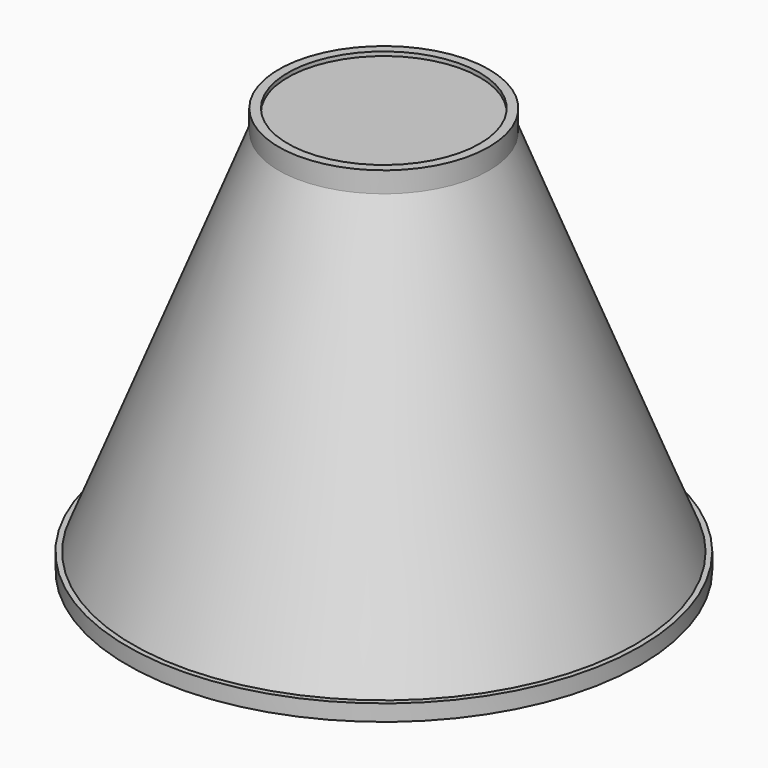
from build123d import *


# Not quite as in the source:
# - a feature of the source that left no trace in its solid (it failed there, or was rolled back) is left out


with BuildPart() as f1:
    # F0 (on Front) → F1 (revolve)
    with BuildSketch(Plane.XZ):
        with BuildLine():
            Line((11.3937472925, 47.8038191795), (0, 47.8038191795))
            Line((0, 47.8038191795), (0, -6.5516876057))
            add(Edge.make_bspline(
                [(0, -6.5516876057), (6.0146157822, -6.2971422391), (17.4152007991, -5.8146565414), (26.2624737662, -1.8656336954), (30.4421838373, 0)],
                knots=[0, 0, 0, 0, 0.5275708021, 1, 1, 1, 1], degree=3))
            Line((30.4421838373, 0), (30.4421838373, 1.9357798155))
            Line((30.4421838373, 1.9357798155), (29.8244003206, 1.9357798155))
            Line((29.8244003206, 1.9357798155), (12.4743720517, 45.8226278424))
            Line((12.4743720517, 45.8226278424), (12.4743720517, 48.2841059566))
            Line((12.4743720517, 48.2841059566), (11.3937472925, 48.2841059566))
            Line((11.3937472925, 48.2841059566), (11.3937472925, 47.8038191795))
        make_face()
    revolve(axis=Axis((0, 0, 20.6260657869), (0, 0, -1)))


solid = f1.part
